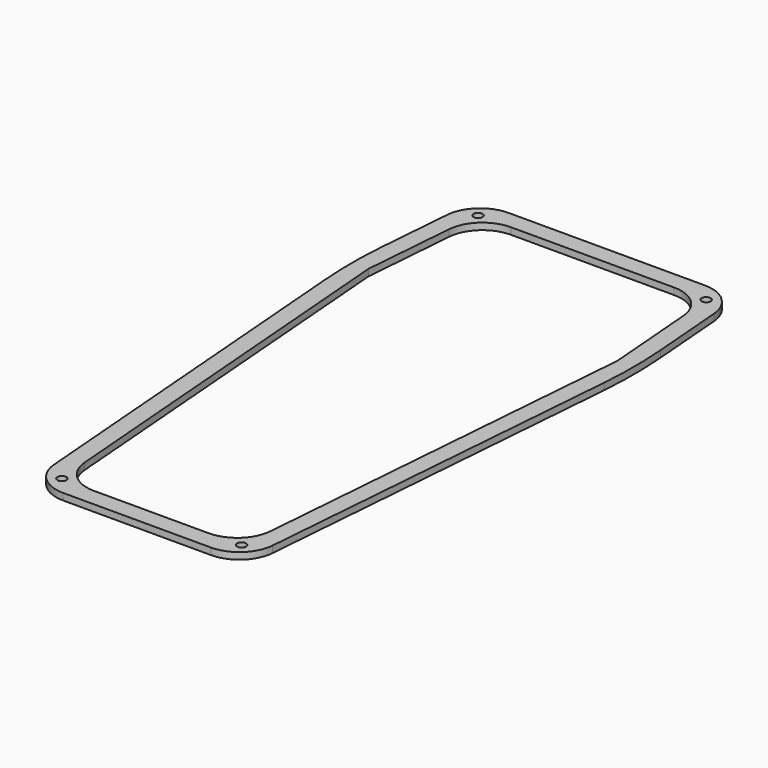
from build123d import *

# Parameters (mm, degrees)
F1_DEPTH = 19.05
F2_R     = 101.6
F3_R     = 1270
F4_R     = 12.827
F5_DEPTH = 19.051


# Not quite as in the source:
# - a feature names something its author has since deleted; it is built from what else it names


with BuildPart() as f1:
    # F0 (on Top) → F1 (new body)
    with BuildSketch(Plane.XY):
        Polygon((-304.8, 0), (0, 0), (304.8, 0), (406.4, 1270), (373.888, 1676.4), (0, 1676.4), (-373.888, 1676.4), (-406.4, 1270), align=None)
        Polygon((-326.989699267, 1625.6), (0, 1625.6), (326.989699267, 1625.6), (355.437699267, 1270), (257.901699267, 50.8), (0, 50.8), (-257.901699267, 50.8), (-355.437699267, 1270), align=None, mode=Mode.SUBTRACT)
    extrude(amount=F1_DEPTH)

    # F2
    f2_edges = [f1.edges().sort_by_distance(p)[0] for p in [
        (-304.8, 0, 9.525),
        (304.8, 0, 9.525),
        (373.888, 1676.4, 9.525),
        (-373.888, 1676.4, 9.525),
        (-326.989699, 1625.6, 9.525),
        (326.989699, 1625.6, 9.525),
        (-257.901699, 50.8, 9.525),
        (257.901699, 50.8, 9.525),
    ]]
    fillet(f2_edges, radius=F2_R)

    # F3
    f3_edges = [f1.edges().sort_by_distance(p)[0] for p in [
        (-406.4, 1270, 9.525),
        (406.4, 1270, 9.525),
    ]]
    fillet(f3_edges, radius=F3_R)

    # F4 (on face) → F5 (cut, through all)
    with BuildSketch(Plane.XY.offset(19.05)):
        with Locations((256.4722616265, 52.3483595568)):
            Circle(F4_R)
        with Locations((-256.4722616265, 52.3483595568)):
            Circle(F4_R)
        with Locations((-325.5602616265, 1624.0516404432)):
            Circle(F4_R)
        with Locations((325.5602616265, 1624.0516404432)):
            Circle(F4_R)
    extrude(amount=-F5_DEPTH, mode=Mode.SUBTRACT)


solid = f1.part
